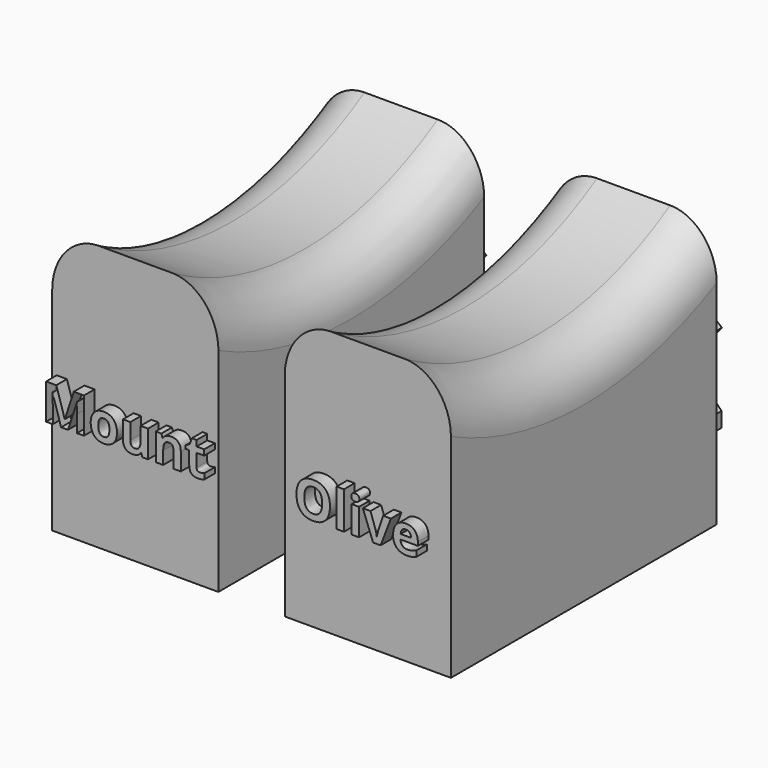
from build123d import *

# Parameters (mm, degrees)
F1_DEPTH      = 50.8
F4_DEPTH      = 76.2
F5_DEPTH      = 76.2
F6_R          = 8.89
F8_TEXT_SIZE  = 9.4116898254
F7_TEXT_SIZE  = 9.4971022621
F9_DEPTH      = 2.54
F10_TEXT_SIZE = 27.1186440678
F11_TEXT_SIZE = 27.0284650173
F12_DEPTH     = 2.54


# Not quite as in the source:
# - Text() gives the source's letters only with a copy of the font that has no kerning and outlines rounded to 1/6400 em; it was checked with that copy


with BuildPart() as f1:
    # F0 (on Top) → F1 (new body)
    with BuildSketch(Plane.XY):
        Polygon((-38.1, 36.83), (-38.1, 5.08), (-38.1, -26.67), (-22.225, -26.67), (-6.35, -26.67), (-6.35, 0), (-6.35, 36.83), (-22.225, 36.83), align=None)
        Polygon((38.1, 36.83), (22.225, 36.83), (6.35, 36.83), (6.35, 0), (6.35, -26.67), (22.225, -26.67), (38.1, -26.67), (38.1, 0), align=None)
    extrude(amount=F1_DEPTH)

    # F3 (on face) → F4 (cut)
    with BuildSketch(Plane(origin=(-38.1, 0, 0), x_dir=(0, -1, 0), z_dir=(-1, 0, 0))):
        with BuildLine():
            Line((26.67, 50.8), (-36.83, 50.8))
            ThreePointArc((-36.83, 50.8), (-5.08, 41.91), (26.67, 50.8))
        make_face()
    extrude(amount=-F4_DEPTH, mode=Mode.SUBTRACT)

    # F2 (on face) → F5 (cut)
    with BuildSketch(Plane.YZ.offset(38.1)):
        with BuildLine():
            Line((36.83, 50.8), (-26.67, 50.8))
            ThreePointArc((-26.67, 50.8), (5.08, 41.91), (36.83, 50.8))
        make_face()
    extrude(amount=-F5_DEPTH, mode=Mode.SUBTRACT)

    # F6
    f6_edges = [f1.edges().sort_by_distance(p)[0] for p in [
        (38.1, 5.08, 41.91),
        (6.35, 5.08, 41.91),
        (-38.1, 5.08, 41.91),
        (-6.35, 5.08, 41.91),
    ]]
    fillet(f6_edges, radius=F6_R)


with BuildPart() as f9:
    # F8 (on face) + F7 (on face) → F9 (new body)
    with BuildSketch(Plane.XZ.offset(26.67)):
        with Locations((10.0646847859, 19.6250434965)):
            Text('Olive', F8_TEXT_SIZE, font='Open Sans', font_style=FontStyle.BOLD, text_align=(TextAlign.LEFT, TextAlign.BOTTOM))
    with BuildSketch(Plane.XZ.offset(26.67)):
        with Locations((-38.1, 19.6244971665)):
            Text('Mount', F7_TEXT_SIZE, font='Open Sans', font_style=FontStyle.BOLD, text_align=(TextAlign.LEFT, TextAlign.BOTTOM))
    extrude(amount=F9_DEPTH)


with BuildPart() as f12:
    # F10 (on face) + F11 (on face) → F12 (new body)
    with BuildSketch(Plane(origin=(0, 36.83, 0), x_dir=(-1, 0, 0), z_dir=(0, 1, 0))):
        with Locations((-38.1, 14.8690417133)):
            Text('20', F10_TEXT_SIZE, font='Open Sans', font_style=FontStyle.BOLD, text_align=(TextAlign.LEFT, TextAlign.BOTTOM))
    with BuildSketch(Plane(origin=(0, 36.83, 0), x_dir=(-1, 0, 0), z_dir=(0, 1, 0))):
        with Locations((6.35, 14.9246028327)):
            Text('17', F11_TEXT_SIZE, font='Open Sans', font_style=FontStyle.BOLD, text_align=(TextAlign.LEFT, TextAlign.BOTTOM))
    extrude(amount=F12_DEPTH)


solid = Compound([f1.part, f9.part, f12.part])
